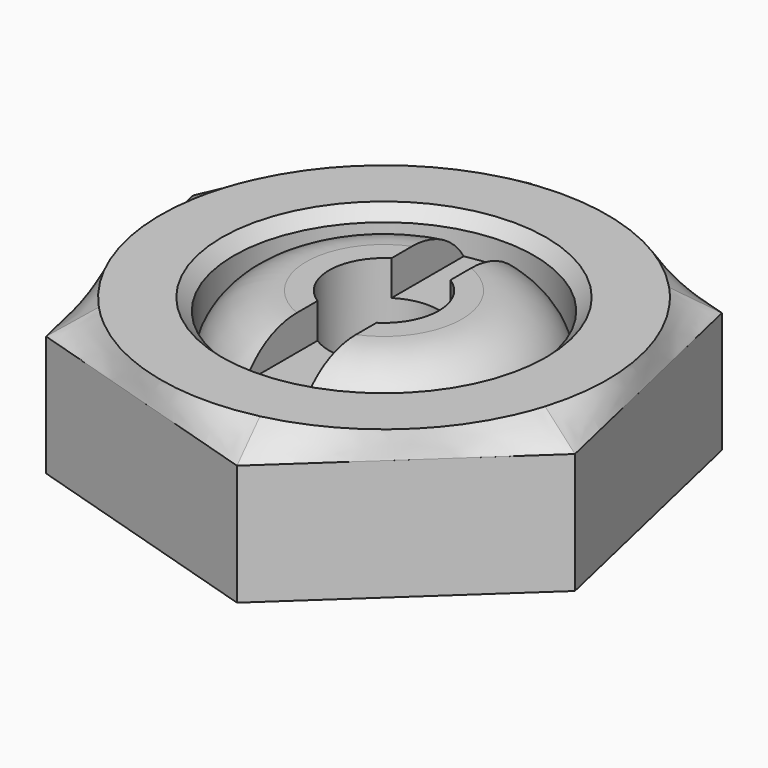
from build123d import *

# Parameters (mm, degrees)
F3_DEPTH  = 2.54
F1_R      = 4.7026824454
F4_DEPTH  = 3.048
F2_R      = 3.1623160727
F6_DEPTH  = 5.08
F7_SIZE   = 0.254
F8_DEPTH  = 3.175
F9_R      = 1.524
F10_W     = 1.2431591749
F10_H     = 6.996748969
F11_DEPTH = 0.7374347188
F12_R     = 1.1551720175
F13_DEPTH = 2.032


# Not quite as in the source:
# - the arcs of a loft's sections are written as splines that run evenly, so that the points pair up as in the source's solid


with BuildPart() as f3:
    # F0 (on Top) → F3 (new body)
    with BuildSketch(Plane.XY):
        Polygon((1.2488487713, -5.4308450613), (5.3276741728, -1.6338877692), (4.0788254014, 3.7969572921), (-1.2488487713, 5.4308450613), (-5.3276741728, 1.6338877692), (-4.0788254014, -3.7969572921), align=None)
    extrude(amount=F3_DEPTH)



with BuildPart() as f4:
    # F1 (on Top) → F4 (new body)
    with BuildSketch(Plane.XY):
        Circle(F1_R)
    extrude(amount=F4_DEPTH)


with BuildPart() as f3_1:
    add(f3.part)

    add(f4.part)  # F5 merges F4
    # F3_face (on face) → F5 section 0
    with BuildSketch(Plane.XY.offset(2.54)):
        Polygon((-5.3276741728, 1.6338877692), (-4.0788254014, -3.7969572921), (1.2488487713, -5.4308450613), (5.3276741728, -1.6338877692), (4.0788254014, 3.7969572921), (-1.2488487713, 5.4308450613), align=None)
    # F4_face (on face) → F5 section 1
    with BuildSketch(Plane.XY.offset(3.048)):
        with BuildLine():
            add(Edge.make_bspline(
                [(-4.4960033295, 1.3788314773), (-4.6564376569, 0.8556977355), (-4.7246126151, 0.30441075), (-4.6682859675, -0.7885026272), (-4.5437982188, -1.3298601483), (-4.1170700938, -2.3375979359), (-3.814934698, -2.8037302861), (-3.4421047517, -3.2042373602)],
                knots=[0, 0, 0, 0, 0.3333333333, 0.3333333333, 0.6666666667, 0.6666666667, 1, 1, 1, 1], degree=3))
            add(Edge.make_bspline(
                [(-3.4421047517, -3.2042373602), (-3.0692748053, -3.6047444343), (-2.6259337502, -3.9394291727), (-1.6512796777, -4.4371055536), (-1.1202064375, -4.5999747613), (-0.0341158506, -4.7342862584), (0.5206343041, -4.7056955053), (1.0538985779, -4.5830688375)],
                knots=[0, 0, 0, 0, 0.3333333333, 0.3333333333, 0.6666666667, 0.6666666667, 1, 1, 1, 1], degree=3))
            add(Edge.make_bspline(
                [(1.0538985779, -4.5830688375), (1.5871628516, -4.4604421698), (2.0986788649, -4.2438399227), (3.0170062898, -3.6486029264), (3.4235917813, -3.270114613), (4.0829542432, -2.3966883224), (4.3355690021, -1.9019652192), (4.4960033295, -1.3788314773)],
                knots=[0, 0, 0, 0, 0.3333333333, 0.3333333333, 0.6666666667, 0.6666666667, 1, 1, 1, 1], degree=3))
            add(Edge.make_bspline(
                [(4.4960033295, -1.3788314773), (4.6564376569, -0.8556977355), (4.7246126151, -0.30441075), (4.6682859675, 0.7885026272), (4.5437982188, 1.3298601483), (4.1170700938, 2.3375979359), (3.814934698, 2.8037302861), (3.4421047517, 3.2042373602)],
                knots=[0, 0, 0, 0, 0.3333333333, 0.3333333333, 0.6666666667, 0.6666666667, 1, 1, 1, 1], degree=3))
            add(Edge.make_bspline(
                [(3.4421047517, 3.2042373602), (3.0692748053, 3.6047444343), (2.6259337502, 3.9394291727), (1.6512796777, 4.4371055536), (1.1202064375, 4.5999747613), (0.0341158506, 4.7342862584), (-0.5206343041, 4.7056955053), (-1.0538985779, 4.5830688375)],
                knots=[0, 0, 0, 0, 0.3333333333, 0.3333333333, 0.6666666667, 0.6666666667, 1, 1, 1, 1], degree=3))
            add(Edge.make_bspline(
                [(-1.0538985779, 4.5830688375), (-1.5871628516, 4.4604421698), (-2.0986788649, 4.2438399227), (-3.0170062898, 3.6486029264), (-3.4235917813, 3.270114613), (-4.0829542432, 2.3966883224), (-4.3355690021, 1.9019652192), (-4.4960033295, 1.3788314773)],
                knots=[0, 0, 0, 0, 0.3333333333, 0.3333333333, 0.6666666667, 0.6666666667, 1, 1, 1, 1], degree=3))
        make_face()
    loft(ruled=True)

    # F2 (on Top) → F6 (cut)
    with BuildSketch(Plane.XY):
        Circle(F2_R)
    extrude(amount=F6_DEPTH, mode=Mode.SUBTRACT)

    # F7
    f7_edges = [f3_1.edges().sort_by_distance(p)[0] for p in [
        (-3.162316, 0, 3.048),
    ]]
    chamfer(f7_edges, length=F7_SIZE)


with BuildPart() as f8:
    # F2 (on Top) → F8 (new body)
    with BuildSketch(Plane.XY):
        Circle(F2_R)
    extrude(amount=F8_DEPTH)

    # F9
    f9_edges = [f8.edges().sort_by_distance(p)[0] for p in [
        (-3.162316, 0, 3.175),
    ]]
    fillet(f9_edges, radius=F9_R)

    # F10 (on face) → F11 (cut)
    with BuildSketch(Plane.XY.offset(3.175)):
        Rectangle(F10_W, F10_H)
    extrude(amount=-F11_DEPTH, mode=Mode.SUBTRACT)

    # F12 (on face) → F13 (cut)
    with BuildSketch(Plane.XY.offset(3.175)):
        Circle(F12_R)
    extrude(amount=-F13_DEPTH, mode=Mode.SUBTRACT)


solid = Compound([f3_1.part, f8.part])
